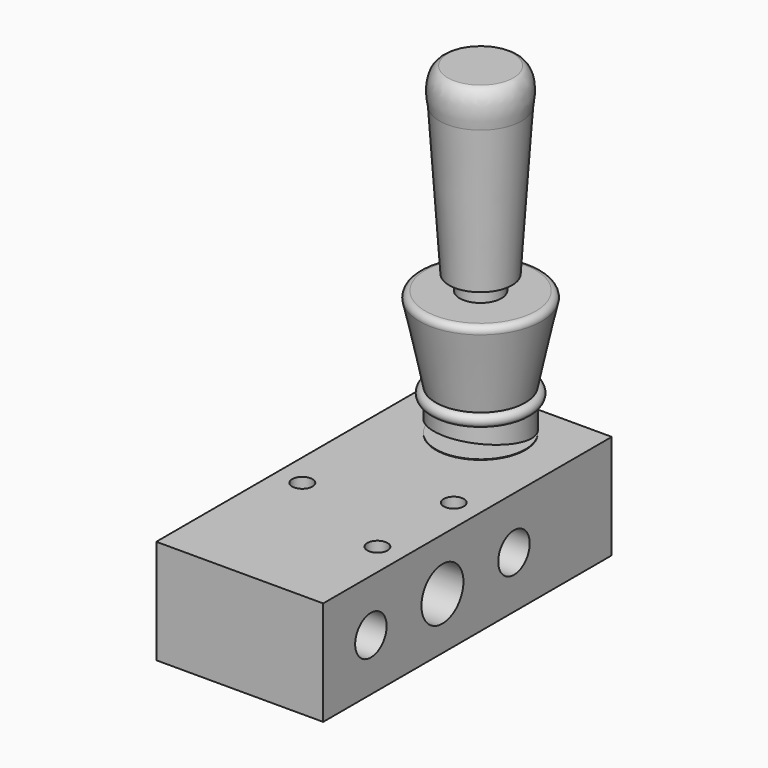
from build123d import *

# Parameters (mm, degrees)
F2_W          = 35.56
F2_H          = 76.835
F3_DEPTH      = 22.225
F4_R          = 4.191
F4_R_2        = 5.588
F6_DEPTH      = 25.4
F5_R          = 5.588
F7_DEPTH      = 25.4
F9_DEPTH      = 17.781
F9_DEPTH_BACK = 17.781
F10_R         = 9.525
F11_DEPTH     = 0.127
F12_R         = 2.159
F13_DEPTH     = 22.226


with BuildPart() as f1:
    # F0 (on Front) → F1 (revolve)
    with BuildSketch(Plane.XZ):
        with BuildLine():
            Line((0, 68.961), (0, 0))
            Line((0, 0), (9.525, 0))
            Line((9.525, 0), (9.525, 6.35))
            ThreePointArc((9.525, 6.35), (10.795, 7.62), (9.525, 8.89))
            Line((9.525, 8.89), (13.0085538918, 25.2627032915))
            ThreePointArc((13.0085538918, 25.2627032915), (12.7534147859, 26.3261380295), (11.766359362, 26.797))
            Line((11.766359362, 26.797), (4.445, 26.797))
            Line((4.445, 26.797), (4.445, 29.972))
            Line((4.445, 29.972), (6.6802, 29.972))
            Line((6.6802, 29.972), (8.763, 61.4476334416))
            add(Edge.make_bspline(
                [(8.763, 61.4476334416), (10.233264787, 68.2599443036), (6.985, 68.961)],
                knots=[4.7123889804, 4.7123889804, 4.7123889804, 6.2831853072, 6.2831853072, 6.2831853072], degree=2, weights=[1, 0.7071067812, 1]))
            Line((6.985, 68.961), (0, 68.961))
        make_face()
    revolve(axis=Axis((0, 0, 34.4805), (0, 0, 1)))

    # F8 (on Right) → F9 (cut, two sides)
    with BuildSketch(Plane.YZ) as f9_sk:
        Polygon((-9.525, 0), (9.525, 0), (-9.525, 3.3590289825), align=None)
    extrude(amount=-F9_DEPTH, mode=Mode.SUBTRACT)
    extrude(f9_sk.sketch, amount=F9_DEPTH_BACK, mode=Mode.SUBTRACT)


with BuildPart() as f3:
    # F2 (on Top) → F3 (new body)
    with BuildSketch(Plane.XY):
        with Locations((0, -25.7175)):
            Rectangle(F2_W, F2_H)
    extrude(amount=-F3_DEPTH)

    # F4 (on face) → F6 (cut)
    with BuildSketch(Plane.YZ.offset(17.78)):
        with Locations((-51.435, -11.1125)):
            Circle(F4_R)
        with Locations((-32.385, -11.1125)):
            Circle(F4_R_2)
        with Locations((-13.335, -11.1125)):
            Circle(F4_R)
    extrude(amount=-F6_DEPTH, mode=Mode.SUBTRACT)

    # F5 (on face) → F7 (cut)
    with BuildSketch(Plane(origin=(-17.78, 0, 0), x_dir=(0, -1, 0), z_dir=(-1, 0, 0))):
        with Locations((45.085, -11.1125)):
            Circle(F5_R)
        with Locations((19.685, -11.1125)):
            Circle(F5_R)
    extrude(amount=-F7_DEPTH, mode=Mode.SUBTRACT)

    # F10 (on face) → F11 (join)
    with BuildSketch(Plane.XY):
        Circle(F10_R)
    extrude(amount=F11_DEPTH)

    # F12 (on face) → F13 (cut, through all)
    with BuildSketch(Plane.XY):
        with Locations((-12.065, -32.385)):
            Circle(F12_R)
        with Locations((12.065, -22.225)):
            Circle(F12_R)
        with Locations((12.065, -42.545)):
            Circle(F12_R)
    extrude(amount=-F13_DEPTH, mode=Mode.SUBTRACT)


solid = Compound([f1.part, f3.part])
